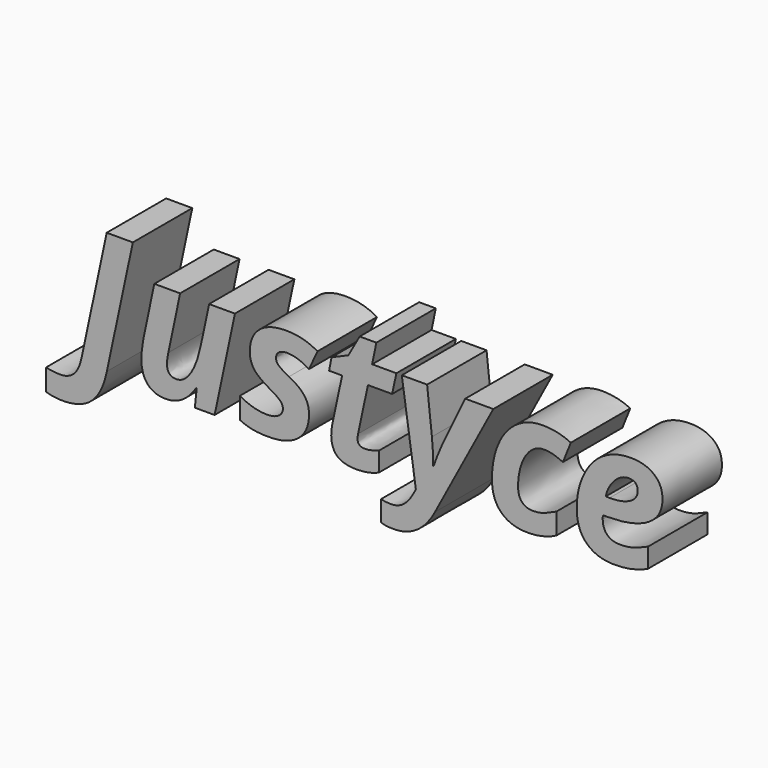
from build123d import *

# Parameters (mm, degrees)
F0_TEXT_SIZE = 30.019548851
F1_DEPTH     = 12.7


# Not quite as in the source:
# - Text() gives the source's letters only with a copy of the font that has no kerning and outlines rounded to 1/6400 em; it was checked with that copy


with BuildPart() as f1:
    # F0 (on Front) → F1 (new body)
    with BuildSketch(Plane.XZ):
        with Locations((-64.9370253086, 4.0763388388)):
            Text('Justyce', F0_TEXT_SIZE, font='Open Sans', font_style=FontStyle.BOLDITALIC, text_align=(TextAlign.LEFT, TextAlign.BOTTOM))
    extrude(amount=F1_DEPTH)


solid = f1.part
